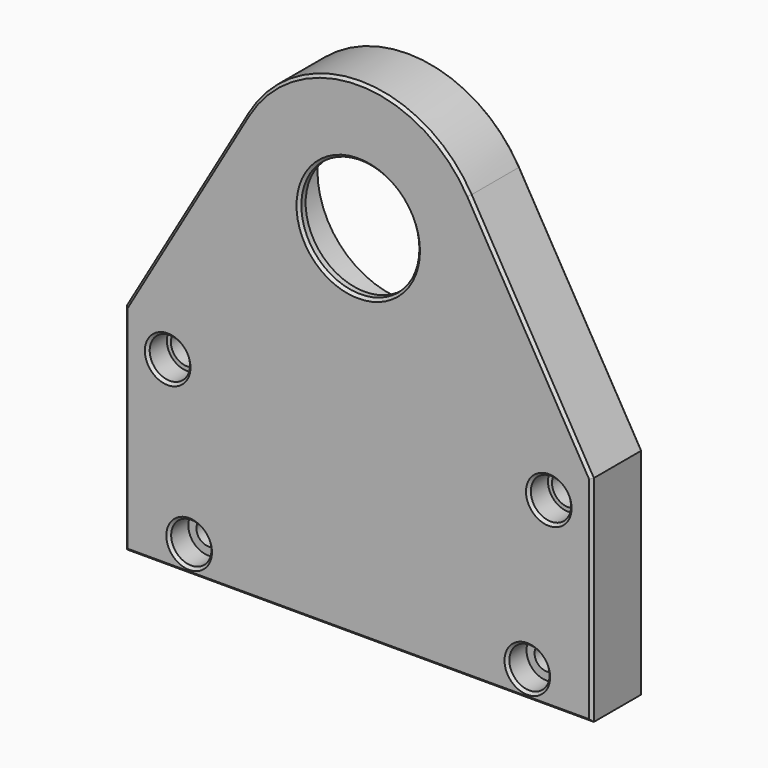
from build123d import *

# Parameters (mm, degrees)
F0_R      = 11
F0_W      = 87
F0_H      = 40
F0_R_2    = 3.75
F0_R_3    = 3
F0_R_4    = 2.25
F1_DEPTH  = 12
F2_R      = 3.75
F2_R_2    = 3
F2_R_3    = 2.25
F3_DEPTH  = 4.5
F4_R      = 20
F5_DEPTH  = 0.5
F6_R      = 16.5
F7_DEPTH  = 1.5
F8_R      = 16
F9_DEPTH  = 9
F10_R     = 13
F11_DEPTH = 10.5
F12_SIZE2 = 0.5
F12_SIZE  = 0.5
F13_SIZE2 = 0.49999
F13_SIZE  = 0.49999
F14_SIZE2 = 0.99999
F14_SIZE  = 0.99999


# Not quite as in the source:
# - a fillet or chamfer is up to 0.001 mm smaller than in the source, because OpenCascade refuses the exact size


with BuildPart() as f1:
    # F0 (on Front) → F1 (new body)
    with BuildSketch(Plane.XZ):
        with BuildLine():
            Line((-43.5, 20), (43.5, 20))
            Line((43.5, 20), (20.7387457553, 59.0790903836))
            ThreePointArc((20.7387457553, 59.0790903836), (0, 71), (-20.7387457553, 59.0790903836))
            Line((-20.7387457553, 59.0790903836), (-43.5, 20))
        make_face()
        with Locations((0, 47)):
            Circle(F0_R, mode=Mode.SUBTRACT)
        Rectangle(F0_W, F0_H)
        with Locations((-31.5, -15)):
            Circle(F0_R_2, mode=Mode.SUBTRACT)
        with Locations((-35.5, 14)):
            Circle(F0_R_2, mode=Mode.SUBTRACT)
        with Locations((31.5, -15)):
            Circle(F0_R_2, mode=Mode.SUBTRACT)
        with Locations((35.5, 14)):
            Circle(F0_R_2, mode=Mode.SUBTRACT)
        with Locations((-35.5, 14)):
            Circle(F0_R_2)
        with Locations((-35.5, 14)):
            Circle(F0_R_3, mode=Mode.SUBTRACT)
        with Locations((-31.5, -15)):
            Circle(F0_R_2)
        with Locations((-31.5, -15)):
            Circle(F0_R_4, mode=Mode.SUBTRACT)
        with Locations((35.5, 14)):
            Circle(F0_R_2)
        with Locations((35.5, 14)):
            Circle(F0_R_3, mode=Mode.SUBTRACT)
        with Locations((31.5, -15)):
            Circle(F0_R_2)
        with Locations((31.5, -15)):
            Circle(F0_R_4, mode=Mode.SUBTRACT)
    extrude(amount=F1_DEPTH)

    # F2 (on face) → F3 (cut)
    with BuildSketch(Plane.XZ.offset(12)):
        with Locations((-35.5, 14)):
            Circle(F2_R)
        with Locations((-35.5, 14)):
            Circle(F2_R_2, mode=Mode.SUBTRACT)
        with Locations((35.5, 14)):
            Circle(F2_R)
        with Locations((35.5, 14)):
            Circle(F2_R_2, mode=Mode.SUBTRACT)
        with Locations((-31.5, -15)):
            Circle(F2_R)
        with Locations((-31.5, -15)):
            Circle(F2_R_3, mode=Mode.SUBTRACT)
        with Locations((31.5, -15)):
            Circle(F2_R)
        with Locations((31.5, -15)):
            Circle(F2_R_3, mode=Mode.SUBTRACT)
    extrude(amount=-F3_DEPTH, mode=Mode.SUBTRACT)

    # F4 (on face) → F5 (cut)
    with BuildSketch(Plane(origin=(0, 0, 0), x_dir=(-1, 0, 0), z_dir=(0, 1, 0))):
        with Locations((0, 47)):
            Circle(F4_R)
    extrude(amount=-F5_DEPTH, mode=Mode.SUBTRACT)

    # F6 (on face) → F7 (cut)
    with BuildSketch(Plane(origin=(0, 0, 0), x_dir=(-1, 0, 0), z_dir=(0, 1, 0))):
        with Locations((0, 47)):
            Circle(F6_R)
    extrude(amount=-F7_DEPTH, mode=Mode.SUBTRACT)

    # F8 (on face) → F9 (cut)
    with BuildSketch(Plane(origin=(0, 0, 0), x_dir=(-1, 0, 0), z_dir=(0, 1, 0))):
        with Locations((0, 47)):
            Circle(F8_R)
    extrude(amount=-F9_DEPTH, mode=Mode.SUBTRACT)

    # F10 (on face) → F11 (cut)
    with BuildSketch(Plane(origin=(0, 0, 0), x_dir=(-1, 0, 0), z_dir=(0, 1, 0))):
        with Locations((0, 47)):
            Circle(F10_R)
    extrude(amount=-F11_DEPTH, mode=Mode.SUBTRACT)

    # F12
    f12_edges = [f1.edges().sort_by_distance(p)[0] for p in [
        (-32.119373, -12, 39.539545),
        (0, -12, 71),
        (-43.5, -12, 0),
        (32.119373, -12, 39.539545),
        (0, -12, -20),
        (43.5, -12, 0),
        (-35.25, -12, -15),
        (-39.25, -12, 14),
        (27.75, -12, -15),
        (31.75, -12, 14),
        (-11, -12, 47),
    ]]
    chamfer(f12_edges, length=F12_SIZE, length2=F12_SIZE2)

    # F13 (size 0.5 and 0.5 in the source; OpenCascade refuses exactly that, so slightly less here)
    f13_edges = [f1.edges().sort_by_distance(p)[0] for p in [
        (-32.119373, 0, 39.539545),
        (0, 0, 71),
        (-43.5, 0, 0),
        (32.119373, 0, 39.539545),
        (0, 0, -20),
        (43.5, 0, 0),
        (-33.75, 0, -15),
        (-38.5, 0, 14),
        (29.25, 0, -15),
        (32.5, 0, 14),
        (20, 0, 47),
    ]]
    chamfer(f13_edges, length=F13_SIZE, length2=F13_SIZE2)

    # F14 (size 1 and 1 in the source; OpenCascade refuses exactly that, so slightly less here)
    f14_edges = [f1.edges().sort_by_distance(p)[0] for p in [
        (16.5, -0.5, 47),
    ]]
    chamfer(f14_edges, length=F14_SIZE, length2=F14_SIZE2)


solid = f1.part
